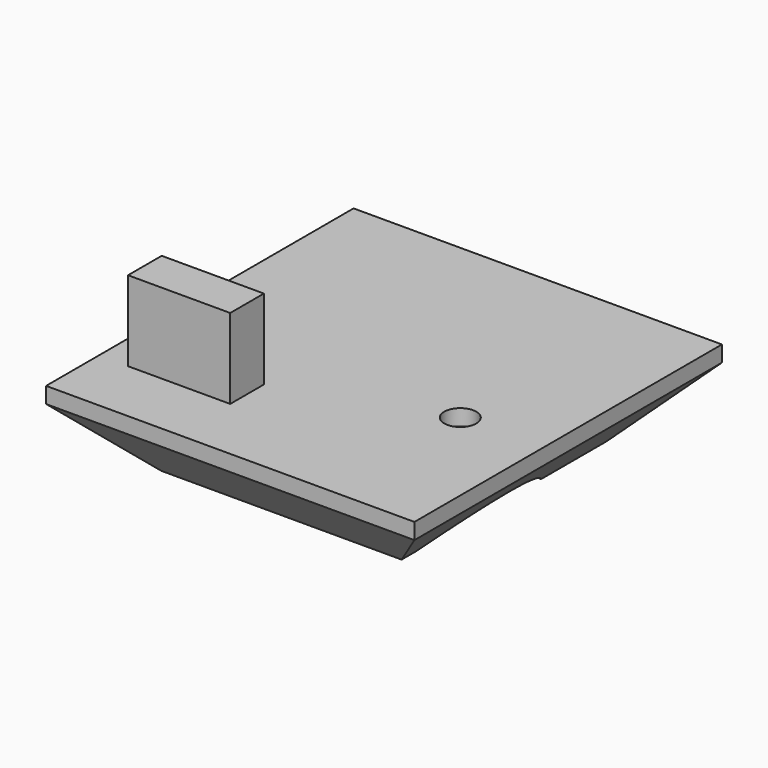
from build123d import *

# Parameters (mm, degrees)
F0_W        = 115
F0_H        = 120
F0_R        = 5
F1_DEPTH    = 25
F2_W        = 31.9062322378
F2_H        = 13.1420847028
F3_DEPTH    = 25
F4_T1_DEPTH = 217.8673195186
F4_T3_DEPTH = 222.8673195186


# Not quite as in the source:
# - a fillet or chamfer that OpenCascade refuses, or shapes differently, is made with other operations: its cross-section is extruded or revolved along the edge and cut away or added


with BuildPart() as f1:
    # F0 (on Top) → F1 (new body)
    with BuildSketch(Plane.XY):
        with Locations((-66.8158578873, 10)):
            Rectangle(F0_W, F0_H)
        with Locations((-35, 0)):
            Circle(F0_R, mode=Mode.SUBTRACT)
    extrude(amount=F1_DEPTH)

    # F2 (on face) → F3 (join)
    with BuildSketch(Plane.XY.offset(25)):
        with Locations((-99.2479249835, -22.8444887325)):
            Rectangle(F2_W, F2_H)
    extrude(amount=F3_DEPTH)

    # F4: chamfer of 20 on 5 edges, made by hand

    # F4_s2 → F4_t1 (cut)
    with BuildSketch(Plane.YZ.offset(-175.7495176466)):
        Polygon((-50, 20), (-30, 0), (-50, 0), align=None)
        Polygon((50, 0), (70, 20), (70, 0), align=None)
    extrude(amount=F4_T1_DEPTH, mode=Mode.SUBTRACT)

    # F4_s4 → F4_t3 (cut)
    with BuildSketch(Plane.XZ.offset(-121.4336597593)):
        Polygon((-9.3158578873, 20), (-29.3158578873, 0), (-9.3158578873, 0), align=None)
        Polygon((-124.3158578873, 20), (-104.3158578873, 0), (-124.3158578873, 0), align=None)
    extrude(amount=F4_T3_DEPTH, mode=Mode.SUBTRACT)

    # F4_s5 → F4_t6 (revolve, cut)
    with BuildSketch(Plane.XZ):
        Polygon((-10, 0), (-30, 20), (-30, 0), align=None)
    revolve(axis=Axis((-35, 0, 0), (0, 0, 1)), mode=Mode.SUBTRACT)


solid = f1.part
